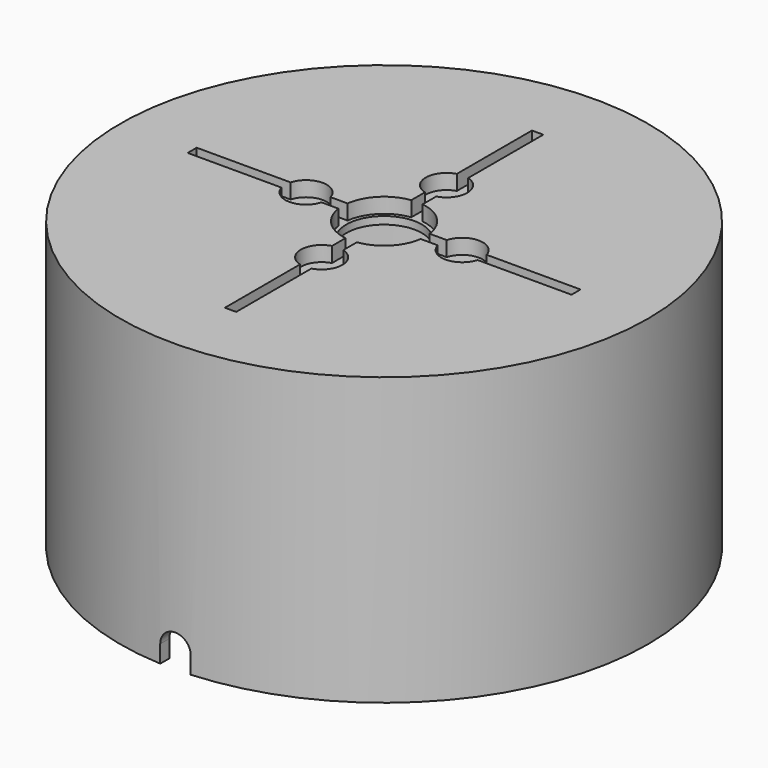
from build123d import *

# Parameters (mm, degrees)
F0_R     = 35
F0_R_2   = 5
F1_DEPTH = 38
F2_DEPTH = 2
F3_R     = 33.5
F4_DEPTH = 35
F5_DEPTH = 38.001
F7_W     = 4
F7_H     = 4.5
F8_DEPTH = 2
F9_R     = 1.999


# Not quite as in the source:
# - a fillet or chamfer is up to 0.001 mm smaller than in the source, because OpenCascade refuses the exact size


with BuildPart() as f1:
    # F0 (on Top) → F1 (new body)
    with BuildSketch(Plane.XY):
        Circle(F0_R)
        with BuildLine():
            ThreePointArc((0.75, 5.4486236794), (3.8890872965, 3.8890872965), (5.4486236794, 0.75))
            Line((5.4486236794, 0.75), (7.7042486889, 0.75))
            ThreePointArc((7.7042486889, 0.75), (10.35, 2.75), (12.9957513111, 0.75))
            Line((12.9957513111, 0.75), (25.4486236794, 0.75))
            Line((25.4486236794, 0.75), (25.4486236794, -0.75))
            Line((25.4486236794, -0.75), (12.9957513111, -0.75))
            ThreePointArc((12.9957513111, -0.75), (10.35, -2.75), (7.7042486889, -0.75))
            Line((7.7042486889, -0.75), (5.4486236794, -0.75))
            ThreePointArc((5.4486236794, -0.75), (3.8890872965, -3.8890872965), (0.75, -5.4486236794))
            Line((0.75, -5.4486236794), (0.75, -7.7042486889))
            ThreePointArc((0.75, -7.7042486889), (2.1937410968, -8.6916876048), (2.75, -10.35))
            ThreePointArc((2.75, -10.35), (2.1937410968, -12.0083123952), (0.75, -12.9957513111))
            Line((0.75, -12.9957513111), (0.75, -25.4486236794))
            Line((0.75, -25.4486236794), (-0.75, -25.4486236794))
            Line((-0.75, -25.4486236794), (-0.75, -12.9957513111))
            ThreePointArc((-0.75, -12.9957513111), (-2.75, -10.35), (-0.75, -7.7042486889))
            Line((-0.75, -7.7042486889), (-0.75, -5.4486236794))
            ThreePointArc((-0.75, -5.4486236794), (-3.8890872965, -3.8890872965), (-5.4486236794, -0.75))
            Line((-5.4486236794, -0.75), (-7.7042486889, -0.75))
            ThreePointArc((-7.7042486889, -0.75), (-10.35, -2.75), (-12.9957513111, -0.75))
            Line((-12.9957513111, -0.75), (-25.4486236794, -0.75))
            Line((-25.4486236794, -0.75), (-25.4486236794, 0.75))
            Line((-25.4486236794, 0.75), (-12.9957513111, 0.75))
            ThreePointArc((-12.9957513111, 0.75), (-10.35, 2.75), (-7.7042486889, 0.75))
            Line((-7.7042486889, 0.75), (-5.4486236794, 0.75))
            ThreePointArc((-5.4486236794, 0.75), (-3.8890872965, 3.8890872965), (-0.75, 5.4486236794))
            Line((-0.75, 5.4486236794), (-0.75, 7.7042486889))
            ThreePointArc((-0.75, 7.7042486889), (-2.75, 10.35), (-0.75, 12.9957513111))
            Line((-0.75, 12.9957513111), (-0.75, 25.4486236794))
            Line((-0.75, 25.4486236794), (0.75, 25.4486236794))
            Line((0.75, 25.4486236794), (0.75, 12.9957513111))
            ThreePointArc((0.75, 12.9957513111), (2.1937410968, 12.0083123952), (2.75, 10.35))
            ThreePointArc((2.75, 10.35), (2.1937410968, 8.6916876048), (0.75, 7.7042486889))
            Line((0.75, 7.7042486889), (0.75, 5.4486236794))
        make_face(mode=Mode.SUBTRACT)
        with BuildLine():
            Line((0.75, -12.9957513111), (0.75, -7.7042486889))
            ThreePointArc((0.75, -7.7042486889), (0, -7.6), (-0.75, -7.7042486889))
            Line((-0.75, -7.7042486889), (-0.75, -12.9957513111))
            ThreePointArc((-0.75, -12.9957513111), (0, -13.1), (0.75, -12.9957513111))
        make_face()
        with BuildLine():
            Line((12.9957513111, 0.75), (7.7042486889, 0.75))
            ThreePointArc((7.7042486889, 0.75), (7.6, 0), (7.7042486889, -0.75))
            Line((7.7042486889, -0.75), (12.9957513111, -0.75))
            ThreePointArc((12.9957513111, -0.75), (13.0738131457, -0.3786052658), (13.1, 0))
            ThreePointArc((13.1, 0), (13.0738131457, 0.3786052658), (12.9957513111, 0.75))
        make_face()
        with BuildLine():
            ThreePointArc((-5.4486236794, -0.75), (-5.5, 0), (-5.4486236794, 0.75))
            Line((-5.4486236794, 0.75), (-7.7042486889, 0.75))
            ThreePointArc((-7.7042486889, 0.75), (-7.6261868543, 0.3786052658), (-7.6, 0))
            ThreePointArc((-7.6, 0), (-7.6261868543, -0.3786052658), (-7.7042486889, -0.75))
            Line((-7.7042486889, -0.75), (-5.4486236794, -0.75))
        make_face()
        with BuildLine():
            Line((-12.9957513111, 0.75), (-7.7042486889, 0.75))
            ThreePointArc((-7.7042486889, 0.75), (-10.35, 2.75), (-12.9957513111, 0.75))
        make_face()
        with BuildLine():
            ThreePointArc((-0.75, 12.9957513111), (0, 13.1), (0.75, 12.9957513111))
            Line((0.75, 12.9957513111), (0.75, 25.4486236794))
            Line((0.75, 25.4486236794), (-0.75, 25.4486236794))
            Line((-0.75, 25.4486236794), (-0.75, 12.9957513111))
        make_face()
        with BuildLine():
            ThreePointArc((-12.9957513111, -0.75), (-10.35, -2.75), (-7.7042486889, -0.75))
            Line((-7.7042486889, -0.75), (-12.9957513111, -0.75))
        make_face()
        with BuildLine():
            ThreePointArc((-12.9957513111, -0.75), (-13.1, 0), (-12.9957513111, 0.75))
            Line((-12.9957513111, 0.75), (-25.4486236794, 0.75))
            Line((-25.4486236794, 0.75), (-25.4486236794, -0.75))
            Line((-25.4486236794, -0.75), (-12.9957513111, -0.75))
        make_face()
        with BuildLine():
            Line((-0.75, -12.9957513111), (-0.75, -7.7042486889))
            ThreePointArc((-0.75, -7.7042486889), (-2.75, -10.35), (-0.75, -12.9957513111))
        make_face()
        with BuildLine():
            Line((0.75, -25.4486236794), (0.75, -12.9957513111))
            ThreePointArc((0.75, -12.9957513111), (0, -13.1), (-0.75, -12.9957513111))
            Line((-0.75, -12.9957513111), (-0.75, -25.4486236794))
            Line((-0.75, -25.4486236794), (0.75, -25.4486236794))
        make_face()
        with BuildLine():
            ThreePointArc((2.75, -10.35), (2.1937410968, -8.6916876048), (0.75, -7.7042486889))
            Line((0.75, -7.7042486889), (0.75, -12.9957513111))
            ThreePointArc((0.75, -12.9957513111), (2.1937410968, -12.0083123952), (2.75, -10.35))
        make_face()
        with BuildLine():
            Line((12.9957513111, -0.75), (7.7042486889, -0.75))
            ThreePointArc((7.7042486889, -0.75), (10.35, -2.75), (12.9957513111, -0.75))
        make_face()
        with BuildLine():
            Line((25.4486236794, 0.75), (12.9957513111, 0.75))
            ThreePointArc((12.9957513111, 0.75), (13.0738131457, 0.3786052658), (13.1, 0))
            ThreePointArc((13.1, 0), (13.0738131457, -0.3786052658), (12.9957513111, -0.75))
            Line((12.9957513111, -0.75), (25.4486236794, -0.75))
            Line((25.4486236794, -0.75), (25.4486236794, 0.75))
        make_face()
        with BuildLine():
            ThreePointArc((5.4486236794, -0.75), (5.4871408874, -0.3758788124), (5.5, 0))
            ThreePointArc((5.5, 0), (5.4871408874, 0.3758788124), (5.4486236794, 0.75))
            ThreePointArc((5.4486236794, 0.75), (3.8890872965, 3.8890872965), (0.75, 5.4486236794))
            ThreePointArc((0.75, 5.4486236794), (0, 5.5), (-0.75, 5.4486236794))
            ThreePointArc((-0.75, 5.4486236794), (-3.8890872965, 3.8890872965), (-5.4486236794, 0.75))
            ThreePointArc((-5.4486236794, 0.75), (-5.5, 0), (-5.4486236794, -0.75))
            ThreePointArc((-5.4486236794, -0.75), (-3.8890872965, -3.8890872965), (-0.75, -5.4486236794))
            ThreePointArc((-0.75, -5.4486236794), (0, -5.5), (0.75, -5.4486236794))
            ThreePointArc((0.75, -5.4486236794), (3.8890872965, -3.8890872965), (5.4486236794, -0.75))
        make_face()
        Circle(F0_R_2, mode=Mode.SUBTRACT)
        with BuildLine():
            ThreePointArc((12.9957513111, 0.75), (10.35, 2.75), (7.7042486889, 0.75))
            Line((7.7042486889, 0.75), (12.9957513111, 0.75))
        make_face()
        with BuildLine():
            ThreePointArc((-0.75, 7.7042486889), (0, 7.6), (0.75, 7.7042486889))
            Line((0.75, 7.7042486889), (0.75, 12.9957513111))
            ThreePointArc((0.75, 12.9957513111), (0, 13.1), (-0.75, 12.9957513111))
            Line((-0.75, 12.9957513111), (-0.75, 7.7042486889))
        make_face()
        with BuildLine():
            ThreePointArc((5.4486236794, 0.75), (5.4871408874, 0.3758788124), (5.5, 0))
            ThreePointArc((5.5, 0), (5.4871408874, -0.3758788124), (5.4486236794, -0.75))
            Line((5.4486236794, -0.75), (7.7042486889, -0.75))
            ThreePointArc((7.7042486889, -0.75), (7.6, 0), (7.7042486889, 0.75))
            Line((7.7042486889, 0.75), (5.4486236794, 0.75))
        make_face()
        with BuildLine():
            Line((0.75, -7.7042486889), (0.75, -5.4486236794))
            ThreePointArc((0.75, -5.4486236794), (0, -5.5), (-0.75, -5.4486236794))
            Line((-0.75, -5.4486236794), (-0.75, -7.7042486889))
            ThreePointArc((-0.75, -7.7042486889), (0, -7.6), (0.75, -7.7042486889))
        make_face()
        with BuildLine():
            ThreePointArc((-0.75, 5.4486236794), (0, 5.5), (0.75, 5.4486236794))
            Line((0.75, 5.4486236794), (0.75, 7.7042486889))
            ThreePointArc((0.75, 7.7042486889), (0, 7.6), (-0.75, 7.7042486889))
            Line((-0.75, 7.7042486889), (-0.75, 5.4486236794))
        make_face()
        Circle(F0_R_2)
        with BuildLine():
            ThreePointArc((-0.75, 12.9957513111), (-2.75, 10.35), (-0.75, 7.7042486889))
            Line((-0.75, 7.7042486889), (-0.75, 12.9957513111))
        make_face()
        with BuildLine():
            Line((0.75, 12.9957513111), (0.75, 7.7042486889))
            ThreePointArc((0.75, 7.7042486889), (2.1937410968, 8.6916876048), (2.75, 10.35))
            ThreePointArc((2.75, 10.35), (2.1937410968, 12.0083123952), (0.75, 12.9957513111))
        make_face()
        with BuildLine():
            ThreePointArc((-7.6, 0), (-7.6261868543, 0.3786052658), (-7.7042486889, 0.75))
            Line((-7.7042486889, 0.75), (-12.9957513111, 0.75))
            ThreePointArc((-12.9957513111, 0.75), (-13.1, 0), (-12.9957513111, -0.75))
            Line((-12.9957513111, -0.75), (-7.7042486889, -0.75))
            ThreePointArc((-7.7042486889, -0.75), (-7.6261868543, -0.3786052658), (-7.6, 0))
        make_face()
    extrude(amount=-F1_DEPTH)

    # F0 (on Top) → F2 (cut)
    with BuildSketch(Plane.XY):
        with BuildLine():
            ThreePointArc((-12.9957513111, -0.75), (-10.35, -2.75), (-7.7042486889, -0.75))
            Line((-7.7042486889, -0.75), (-12.9957513111, -0.75))
        make_face()
        with BuildLine():
            Line((-12.9957513111, 0.75), (-7.7042486889, 0.75))
            ThreePointArc((-7.7042486889, 0.75), (-10.35, 2.75), (-12.9957513111, 0.75))
        make_face()
        with BuildLine():
            ThreePointArc((-7.6, 0), (-7.6261868543, 0.3786052658), (-7.7042486889, 0.75))
            Line((-7.7042486889, 0.75), (-12.9957513111, 0.75))
            ThreePointArc((-12.9957513111, 0.75), (-13.1, 0), (-12.9957513111, -0.75))
            Line((-12.9957513111, -0.75), (-7.7042486889, -0.75))
            ThreePointArc((-7.7042486889, -0.75), (-7.6261868543, -0.3786052658), (-7.6, 0))
        make_face()
        with BuildLine():
            ThreePointArc((-12.9957513111, -0.75), (-13.1, 0), (-12.9957513111, 0.75))
            Line((-12.9957513111, 0.75), (-25.4486236794, 0.75))
            Line((-25.4486236794, 0.75), (-25.4486236794, -0.75))
            Line((-25.4486236794, -0.75), (-12.9957513111, -0.75))
        make_face()
        with BuildLine():
            ThreePointArc((-5.4486236794, -0.75), (-5.5, 0), (-5.4486236794, 0.75))
            Line((-5.4486236794, 0.75), (-7.7042486889, 0.75))
            ThreePointArc((-7.7042486889, 0.75), (-7.6261868543, 0.3786052658), (-7.6, 0))
            ThreePointArc((-7.6, 0), (-7.6261868543, -0.3786052658), (-7.7042486889, -0.75))
            Line((-7.7042486889, -0.75), (-5.4486236794, -0.75))
        make_face()
        with BuildLine():
            ThreePointArc((5.4486236794, -0.75), (5.4871408874, -0.3758788124), (5.5, 0))
            ThreePointArc((5.5, 0), (5.4871408874, 0.3758788124), (5.4486236794, 0.75))
            ThreePointArc((5.4486236794, 0.75), (3.8890872965, 3.8890872965), (0.75, 5.4486236794))
            ThreePointArc((0.75, 5.4486236794), (0, 5.5), (-0.75, 5.4486236794))
            ThreePointArc((-0.75, 5.4486236794), (-3.8890872965, 3.8890872965), (-5.4486236794, 0.75))
            ThreePointArc((-5.4486236794, 0.75), (-5.5, 0), (-5.4486236794, -0.75))
            ThreePointArc((-5.4486236794, -0.75), (-3.8890872965, -3.8890872965), (-0.75, -5.4486236794))
            ThreePointArc((-0.75, -5.4486236794), (0, -5.5), (0.75, -5.4486236794))
            ThreePointArc((0.75, -5.4486236794), (3.8890872965, -3.8890872965), (5.4486236794, -0.75))
        make_face()
        Circle(F0_R_2, mode=Mode.SUBTRACT)
        with BuildLine():
            Line((0.75, 12.9957513111), (0.75, 7.7042486889))
            ThreePointArc((0.75, 7.7042486889), (2.1937410968, 8.6916876048), (2.75, 10.35))
            ThreePointArc((2.75, 10.35), (2.1937410968, 12.0083123952), (0.75, 12.9957513111))
        make_face()
        with BuildLine():
            ThreePointArc((-0.75, 12.9957513111), (-2.75, 10.35), (-0.75, 7.7042486889))
            Line((-0.75, 7.7042486889), (-0.75, 12.9957513111))
        make_face()
        with BuildLine():
            ThreePointArc((-0.75, 7.7042486889), (0, 7.6), (0.75, 7.7042486889))
            Line((0.75, 7.7042486889), (0.75, 12.9957513111))
            ThreePointArc((0.75, 12.9957513111), (0, 13.1), (-0.75, 12.9957513111))
            Line((-0.75, 12.9957513111), (-0.75, 7.7042486889))
        make_face()
        with BuildLine():
            ThreePointArc((-0.75, 5.4486236794), (0, 5.5), (0.75, 5.4486236794))
            Line((0.75, 5.4486236794), (0.75, 7.7042486889))
            ThreePointArc((0.75, 7.7042486889), (0, 7.6), (-0.75, 7.7042486889))
            Line((-0.75, 7.7042486889), (-0.75, 5.4486236794))
        make_face()
        with BuildLine():
            ThreePointArc((-0.75, 12.9957513111), (0, 13.1), (0.75, 12.9957513111))
            Line((0.75, 12.9957513111), (0.75, 25.4486236794))
            Line((0.75, 25.4486236794), (-0.75, 25.4486236794))
            Line((-0.75, 25.4486236794), (-0.75, 12.9957513111))
        make_face()
        with BuildLine():
            Line((12.9957513111, 0.75), (7.7042486889, 0.75))
            ThreePointArc((7.7042486889, 0.75), (7.6, 0), (7.7042486889, -0.75))
            Line((7.7042486889, -0.75), (12.9957513111, -0.75))
            ThreePointArc((12.9957513111, -0.75), (13.0738131457, -0.3786052658), (13.1, 0))
            ThreePointArc((13.1, 0), (13.0738131457, 0.3786052658), (12.9957513111, 0.75))
        make_face()
        with BuildLine():
            ThreePointArc((12.9957513111, 0.75), (10.35, 2.75), (7.7042486889, 0.75))
            Line((7.7042486889, 0.75), (12.9957513111, 0.75))
        make_face()
        with BuildLine():
            Line((12.9957513111, -0.75), (7.7042486889, -0.75))
            ThreePointArc((7.7042486889, -0.75), (10.35, -2.75), (12.9957513111, -0.75))
        make_face()
        with BuildLine():
            ThreePointArc((5.4486236794, 0.75), (5.4871408874, 0.3758788124), (5.5, 0))
            ThreePointArc((5.5, 0), (5.4871408874, -0.3758788124), (5.4486236794, -0.75))
            Line((5.4486236794, -0.75), (7.7042486889, -0.75))
            ThreePointArc((7.7042486889, -0.75), (7.6, 0), (7.7042486889, 0.75))
            Line((7.7042486889, 0.75), (5.4486236794, 0.75))
        make_face()
        with BuildLine():
            Line((25.4486236794, 0.75), (12.9957513111, 0.75))
            ThreePointArc((12.9957513111, 0.75), (13.0738131457, 0.3786052658), (13.1, 0))
            ThreePointArc((13.1, 0), (13.0738131457, -0.3786052658), (12.9957513111, -0.75))
            Line((12.9957513111, -0.75), (25.4486236794, -0.75))
            Line((25.4486236794, -0.75), (25.4486236794, 0.75))
        make_face()
        with BuildLine():
            Line((0.75, -25.4486236794), (0.75, -12.9957513111))
            ThreePointArc((0.75, -12.9957513111), (0, -13.1), (-0.75, -12.9957513111))
            Line((-0.75, -12.9957513111), (-0.75, -25.4486236794))
            Line((-0.75, -25.4486236794), (0.75, -25.4486236794))
        make_face()
        with BuildLine():
            Line((0.75, -12.9957513111), (0.75, -7.7042486889))
            ThreePointArc((0.75, -7.7042486889), (0, -7.6), (-0.75, -7.7042486889))
            Line((-0.75, -7.7042486889), (-0.75, -12.9957513111))
            ThreePointArc((-0.75, -12.9957513111), (0, -13.1), (0.75, -12.9957513111))
        make_face()
        with BuildLine():
            Line((-0.75, -12.9957513111), (-0.75, -7.7042486889))
            ThreePointArc((-0.75, -7.7042486889), (-2.75, -10.35), (-0.75, -12.9957513111))
        make_face()
        with BuildLine():
            ThreePointArc((2.75, -10.35), (2.1937410968, -8.6916876048), (0.75, -7.7042486889))
            Line((0.75, -7.7042486889), (0.75, -12.9957513111))
            ThreePointArc((0.75, -12.9957513111), (2.1937410968, -12.0083123952), (2.75, -10.35))
        make_face()
        with BuildLine():
            Line((0.75, -7.7042486889), (0.75, -5.4486236794))
            ThreePointArc((0.75, -5.4486236794), (0, -5.5), (-0.75, -5.4486236794))
            Line((-0.75, -5.4486236794), (-0.75, -7.7042486889))
            ThreePointArc((-0.75, -7.7042486889), (0, -7.6), (0.75, -7.7042486889))
        make_face()
    extrude(amount=-F2_DEPTH, mode=Mode.SUBTRACT)

    # F3 (on face) → F4 (cut)
    with BuildSketch(Plane(origin=(0, 0, -38), x_dir=(1, 0, 0), z_dir=(0, 0, -1))):
        Circle(F3_R)
    extrude(amount=-F4_DEPTH, mode=Mode.SUBTRACT)

    # F0 (on Top) → F5 (cut, through all)
    with BuildSketch(Plane.XY):
        Circle(F0_R_2)
    extrude(amount=-F5_DEPTH, mode=Mode.SUBTRACT)

    # F7 (on offset) → F8 (cut)
    with BuildSketch(Plane.XZ.offset(35)):
        with Locations((0.2834053928, -35.936942324)):
            Rectangle(F7_W, F7_H)
    extrude(amount=-F8_DEPTH, mode=Mode.SUBTRACT)

    # F9 (radius 2 in the source; OpenCascade refuses exactly that, so slightly less here)
    f9_edges = [f1.edges().sort_by_distance(p)[0] for p in [
        (2.283405, -34.173763, -33.686942),
        (-1.716595, -34.206935, -33.686942),
    ]]
    fillet(f9_edges, radius=F9_R)


solid = f1.part
